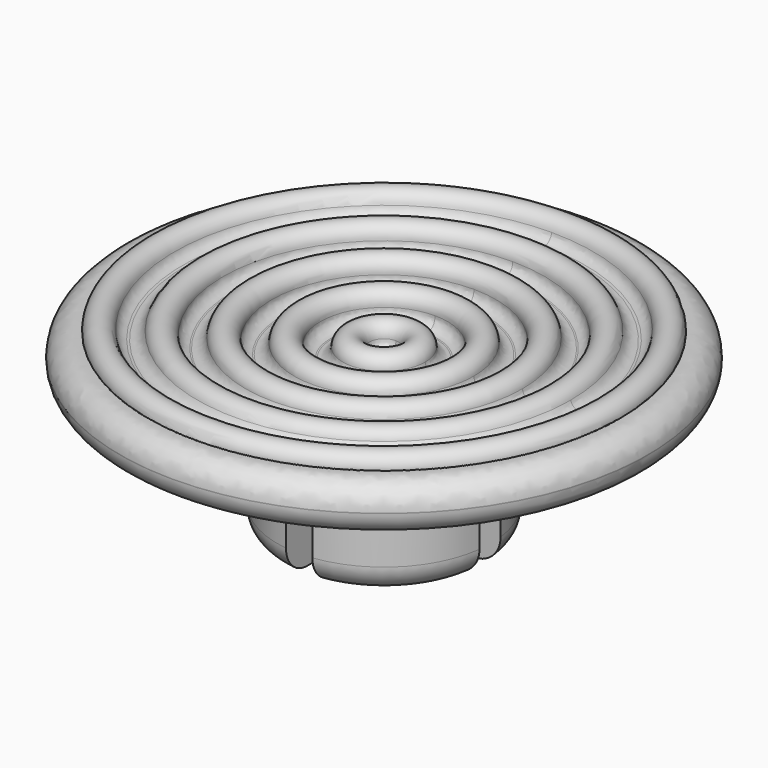
from build123d import *

# Parameters (mm, degrees)
F0_W     = 4.05
F0_H     = 4.5
F2_R     = 0.88
F3_R     = 0.5
F6_R     = 0.4
F7_R     = 0.99999
F9_DEPTH = 3


# Not quite as in the source:
# - a fillet or chamfer is up to 0.001 mm smaller than in the source, because OpenCascade refuses the exact size


with BuildPart() as f1:
    # F0 (on Right) → F1 (revolve)
    with BuildSketch(Plane.YZ):
        Polygon((0, 5), (0, 4.5), (4.05, 4.5), (5.05, 4.5), (5.05, 5), (4, 5), align=None)
        with BuildLine():
            Line((0, 5.8095909261), (0, 5))
            Line((0, 5), (4, 5))
            Line((4, 5), (5.05, 5))
            Line((5.05, 5), (10, 5))
            Line((10, 5), (10, 7))
            ThreePointArc((10, 7), (5.0353022194, 6.1082401009), (0, 5.8095909261))
        make_face()
        with Locations((2.025, 2.25)):
            Rectangle(F0_W, F0_H)
    revolve(axis=Axis((0, 0, 2.25), (0, 0, -1)))

    # F2
    f2_edges = [f1.edges().sort_by_distance(p)[0] for p in [
        (0, -10, 5),
        (0, -10, 7),
        (0, 10, 6),
    ]]
    fillet(f2_edges, radius=F2_R)

    # F3 (on Front) + F0 (on Right) → F4 (revolve)
    with BuildSketch(Plane.XZ):
        with Locations((1.0625054974, 6.2286641949)):
            Circle(F3_R)
        with Locations((2.9060423202, 6.3626512513)):
            Circle(F3_R)
        with Locations((4.7495791431, 6.4966383077)):
            Circle(F3_R)
        with Locations((6.5931159659, 6.6306253641)):
            Circle(F3_R)
        with Locations((8.4366527888, 6.7646124205)):
            Circle(F3_R)
    with BuildSketch(Plane.YZ):
        Polygon((0, 5), (0, 4.5), (4.05, 4.5), (5.05, 4.5), (5.05, 5), (4, 5), align=None)
    revolve(axis=Axis((0, 0, 3.0807434971), (0, 0, -1)))

    # F5: union 

    # F6
    f6_edges = [f1.edges().sort_by_distance(p)[0] for p in [
        (-5.641916, -5.641916, 6.563517),
        (5.641916, 5.641916, 6.563517),
        (4.417067, 4.417067, 6.270099),
        (-4.417067, -4.417067, 6.270099),
        (6.397182, 0, 7.090636),
        (-7.093116, 0, 6.630625),
        (3.584618, 3.584618, 6.112315),
        (-3.584618, -3.584618, 6.112315),
        (-3.19885, -3.19885, 6.050489),
        (3.19885, 3.19885, 6.050489),
        (2.227405, 2.227405, 5.92622),
        (-2.227405, -2.227405, 5.92622),
        (-1.926458, -1.926458, 5.896803),
        (1.926458, 1.926458, 5.896803),
        (0.966091, 0.966091, 5.831507),
        (-0.966091, -0.966091, 5.831507),
        (-0.550931, -0.550931, 5.816717),
        (0.550931, 0.550931, 5.816717),
        (4.973611, 4.973611, 6.394313),
        (-4.973611, -4.973611, 6.394313),
    ]]
    fillet(f6_edges, radius=F6_R)

    # F7 (radius 1 in the source; OpenCascade refuses exactly that, so slightly less here)
    f7_edges = [f1.edges().sort_by_distance(p)[0] for p in [
        (0, -4.05, 4.5),
        (0, -4.05, 0),
    ]]
    fillet(f7_edges, radius=F7_R)

    # F8 (on Top) → F9 (cut)
    with BuildSketch(Plane.XY):
        Polygon((0.5, 0.5), (0.5, 15), (-0.5, 15), (-0.5, 0.5), (-15, 0.5), (-15, -0.5), (-0.5, -0.5), (-0.5, -15), (0.5, -15), (0.5, -0.5), (15, -0.5), (15, 0.5), align=None)
    extrude(amount=F9_DEPTH, mode=Mode.SUBTRACT)


solid = f1.part
